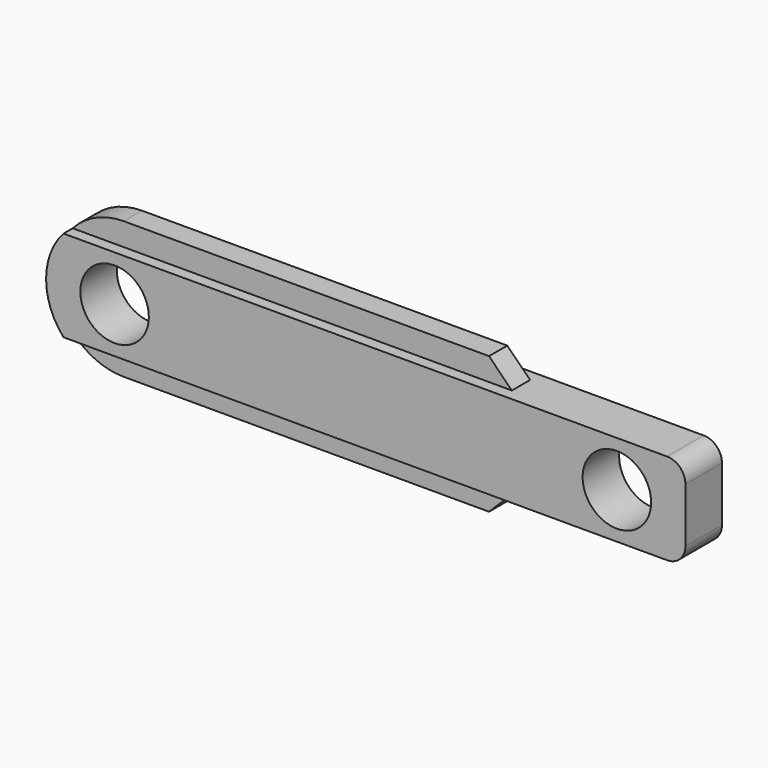
from build123d import *

# Parameters (mm, degrees)
F0_R          = 4.7625
F1_DEPTH      = 6.35
F5_DEPTH      = 1.5875
F5_DEPTH_BACK = 1.5875
F6_SIZE       = 3.17499
F7_R          = 9.52499


# Not quite as in the source:
# - a fillet or chamfer is up to 0.001 mm smaller than in the source, because OpenCascade refuses the exact size


with BuildPart() as f1:
    # F0 (on Front) → F1 (new body)
    with BuildSketch(Plane.XZ):
        with BuildLine():
            ThreePointArc((44.45, 3.81), (43.7060512242, 5.6060512242), (41.91, 6.35))
            Line((41.91, 6.35), (-41.91, 6.35))
            ThreePointArc((-41.91, 6.35), (-43.7060512242, 5.6060512242), (-44.45, 3.81))
            Line((-44.45, 3.81), (-44.45, -3.81))
            ThreePointArc((-44.45, -3.81), (-43.7060512242, -5.6060512242), (-41.91, -6.35))
            Line((-41.91, -6.35), (41.91, -6.35))
            ThreePointArc((41.91, -6.35), (43.7060512242, -5.6060512242), (44.45, -3.81))
            Line((44.45, -3.81), (44.45, 3.81))
        make_face()
        with Locations((-34.925, 0)):
            Circle(F0_R, mode=Mode.SUBTRACT)
        with Locations((34.925, 0)):
            Circle(F0_R, mode=Mode.SUBTRACT)
    extrude(amount=F1_DEPTH)

    # F4 (on face) → F5 (join, two sides)
    with BuildSketch(Plane(origin=(0, -3.175, 0), x_dir=(-1, 0, 0), z_dir=(0, 1, 0))) as f5_sk:
        Polygon((36.3781489432, 5.461), (44.45, 0), (44.45, 9.525), (-19.05, 9.525), (-19.05, 5.461), (29.7344345599, 5.461), align=None)
        Polygon((-19.05, -5.461), (-19.05, -9.525), (44.45, -9.525), (44.45, 0), (36.3781489432, -5.461), (29.7344345599, -5.461), align=None)
    extrude(amount=F5_DEPTH)
    extrude(f5_sk.sketch, amount=-F5_DEPTH_BACK)

    # F6 (size 3.175 in the source; OpenCascade refuses exactly that, so slightly less here)
    f6_edges = [f1.edges().sort_by_distance(p)[0] for p in [
        (19.05, -3.175, 9.525),
        (19.05, -3.175, -9.525),
    ]]
    chamfer(f6_edges, length=F6_SIZE)

    # F7 (radius 9.525 in the source; OpenCascade refuses exactly that, so slightly less here)
    f7_edges = [f1.edges().sort_by_distance(p)[0] for p in [
        (-44.45, -3.175, 9.525),
        (-44.45, -3.175, -9.525),
    ]]
    fillet(f7_edges, radius=F7_R)


solid = f1.part
